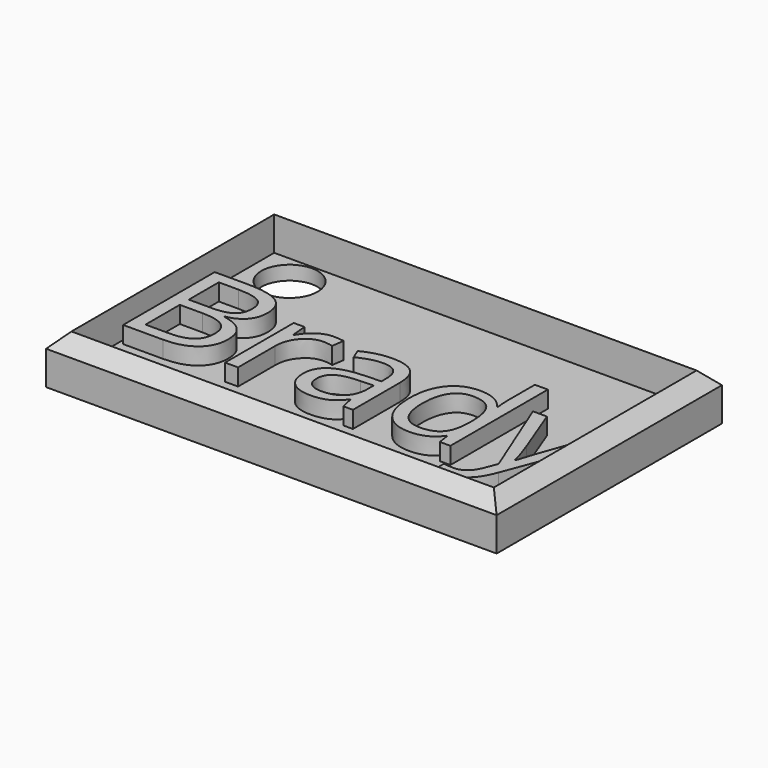
from build123d import *

# Parameters (mm, degrees)
F0_W         = 80
F0_H         = 50
F1_DEPTH     = 11
F2_T         = -2.5
F4_D         = 10
F5_TEXT_SIZE = 28.4679259898
F6_DEPTH     = 3
F7_T1_DEPTH  = 75.7168298797
F7_T3_DEPTH  = 105.7168298797


# Not quite as in the source:
# - a fillet or chamfer that OpenCascade refuses, or shapes differently, is made with other operations: its cross-section is extruded or revolved along the edge and cut away or added
# - Text() gives the source's letters only with a copy of the font that has no kerning and outlines rounded to 1/6400 em; it was checked with that copy


with BuildPart() as f1:
    # F0 (on Top) → F1 (new body)
    with BuildSketch(Plane.XY):
        with Locations((40, -25)):
            Rectangle(F0_W, F0_H)
    extrude(amount=F1_DEPTH)

    # F2
    f2_openings = [f1.faces().sort_by_distance(p)[0] for p in [
        (40, -25, 11),
    ]]
    offset(amount=F2_T, openings=f2_openings)

    # F4 (through all)
    with Locations(Plane.XY.offset(2.5)):
        with Locations((9.5100607723, -7.8558754176)):
            Hole(F4_D / 2)

    # F5 (on face) → F6 (join)
    with BuildSketch(Plane.XY.offset(2.5)):
        with Locations((0.4804013297, -36.9905112311)):
            Text('Brady', F5_TEXT_SIZE, font='Open Sans', text_align=(TextAlign.LEFT, TextAlign.BOTTOM))
    extrude(amount=F6_DEPTH)

    # F7: chamfer of 5 on 4 edges, made by hand

    # F7_s2 → F7_t1 (cut)
    with BuildSketch(Plane.XZ.offset(-12.8584149398)):
        Polygon((0, 6), (5, 11), (0, 11), align=None)
        Polygon((80, 6), (75, 11), (80, 11), align=None)
    extrude(amount=F7_T1_DEPTH, mode=Mode.SUBTRACT)

    # F7_s4 → F7_t3 (cut)
    with BuildSketch(Plane.YZ.offset(-12.8584149398)):
        Polygon((0, 6), (-5, 11), (0, 11), align=None)
        Polygon((-45, 11), (-50, 6), (-50, 11), align=None)
    extrude(amount=F7_T3_DEPTH, mode=Mode.SUBTRACT)


solid = f1.part
